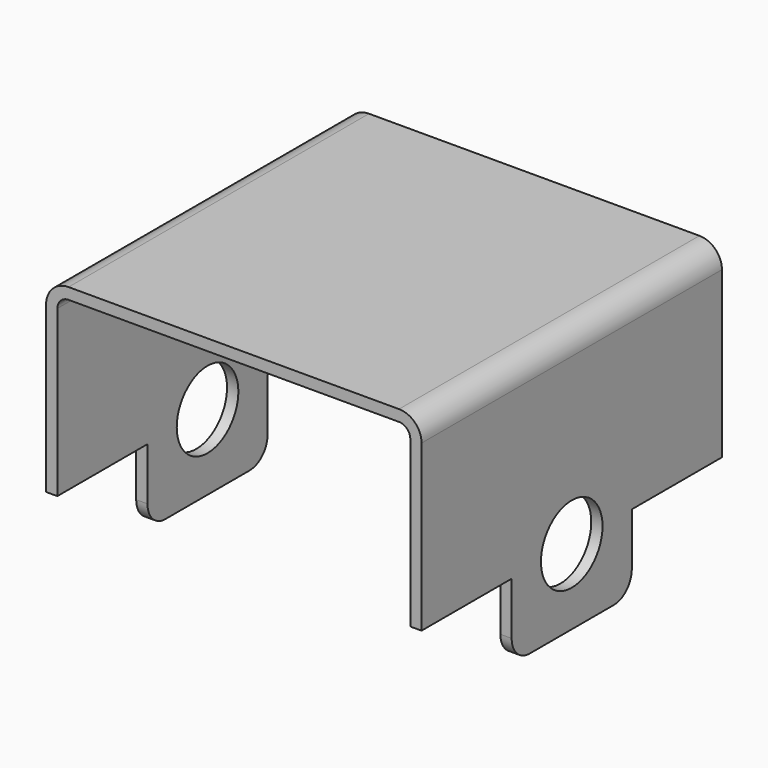
from build123d import *
from build123d import SkipClean  # not in build123d's __all__

# Parameters (mm, degrees)
F1_DEPTH = 100
F3_DEPTH = 3
F4_DEPTH = 3
F6_DEPTH = 3
F7_R     = 10.25
F8_DEPTH = 3


# Not quite as in the source:
# - a feature names something its author has since deleted; it is built from what else it names


with BuildPart() as f1:
    # F0 (on Front) → F1 (new body)
    with BuildSketch(Plane.XZ):
        with BuildLine():
            Line((-44, 20.8545142158), (0, 20.8545142158))
            Line((0, 20.8545142158), (0, 23.8545142158))
            Line((0, 23.8545142158), (-44, 23.8545142158))
            ThreePointArc((-44, 23.8545142158), (-48.2426406871, 22.0971549029), (-50, 17.8545142158))
            Line((-50, 17.8545142158), (-50, -26.1454857842))
            Line((-50, -26.1454857842), (-47, -26.1454857842))
            Line((-47, -26.1454857842), (-47, 17.8545142158))
            ThreePointArc((-47, 17.8545142158), (-46.1213203436, 19.9758345594), (-44, 20.8545142158))
        make_face()
        with BuildLine():
            Line((0, 23.8545142158), (0, 20.8545142158))
            Line((0, 20.8545142158), (44, 20.8545142158))
            ThreePointArc((44, 20.8545142158), (46.1213203436, 19.9758345594), (47, 17.8545142158))
            Line((47, 17.8545142158), (47, -26.1454857842))
            Line((47, -26.1454857842), (50, -26.1454857842))
            Line((50, -26.1454857842), (50, 17.8545142158))
            ThreePointArc((50, 17.8545142158), (48.2426406871, 22.0971549029), (44, 23.8545142158))
            Line((44, 23.8545142158), (0, 23.8545142158))
        make_face()
    extrude(amount=F1_DEPTH)

    # F2 (on face) → F3 (cut)
    with BuildSketch(Plane(origin=(-50, 0, 0), x_dir=(0, -1, 0), z_dir=(-1, 0, 0))):
        with BuildLine():
            Line((39.75, -26.1454857842), (60.25, -26.1454857842))
            ThreePointArc((60.25, -26.1454857842), (50, -15.8954857842), (39.75, -26.1454857842))
        make_face()
    extrude(amount=-F3_DEPTH, mode=Mode.SUBTRACT)

    # F2 (on face) → F4 (join)
    with BuildSketch(Plane(origin=(-50, 0, 0), x_dir=(0, -1, 0), z_dir=(-1, 0, 0))):
        with BuildLine():
            Line((70, -26.1454857842), (60.25, -26.1454857842))
            ThreePointArc((60.25, -26.1454857842), (50, -36.3954857842), (39.75, -26.1454857842))
            Line((39.75, -26.1454857842), (30, -26.1454857842))
            Line((30, -26.1454857842), (30, -40.1454857842))
            ThreePointArc((30, -40.1454857842), (31.7573593129, -44.3881264713), (36, -46.1454857842))
            Line((36, -46.1454857842), (64, -46.1454857842))
            ThreePointArc((64, -46.1454857842), (68.2426406871, -44.3881264713), (70, -40.1454857842))
            Line((70, -40.1454857842), (70, -26.1454857842))
        make_face()
    with SkipClean():  # cleaning this boolean's faces spoils the solid; the shape is the same uncleaned
        extrude(amount=-F4_DEPTH)

    # F5 (on face) → F6 (join)
    with BuildSketch(Plane.YZ.offset(50)):
        with BuildLine():
            Line((-30, -26.1454857842), (-70, -26.1454857842))
            Line((-70, -26.1454857842), (-70, -40.1454857842))
            ThreePointArc((-70, -40.1454857842), (-68.2426406871, -44.3881264713), (-64, -46.1454857842))
            Line((-64, -46.1454857842), (-36, -46.1454857842))
            ThreePointArc((-36, -46.1454857842), (-31.7573593129, -44.3881264713), (-30, -40.1454857842))
            Line((-30, -40.1454857842), (-30, -26.1454857842))
        make_face()
    extrude(amount=-F6_DEPTH)

    # F7 (on face) → F8 (cut)
    with BuildSketch(Plane.YZ.offset(50)):
        with Locations((-50, -26.1454857842)):
            Circle(F7_R)
    extrude(amount=-F8_DEPTH, mode=Mode.SUBTRACT)


solid = f1.part
